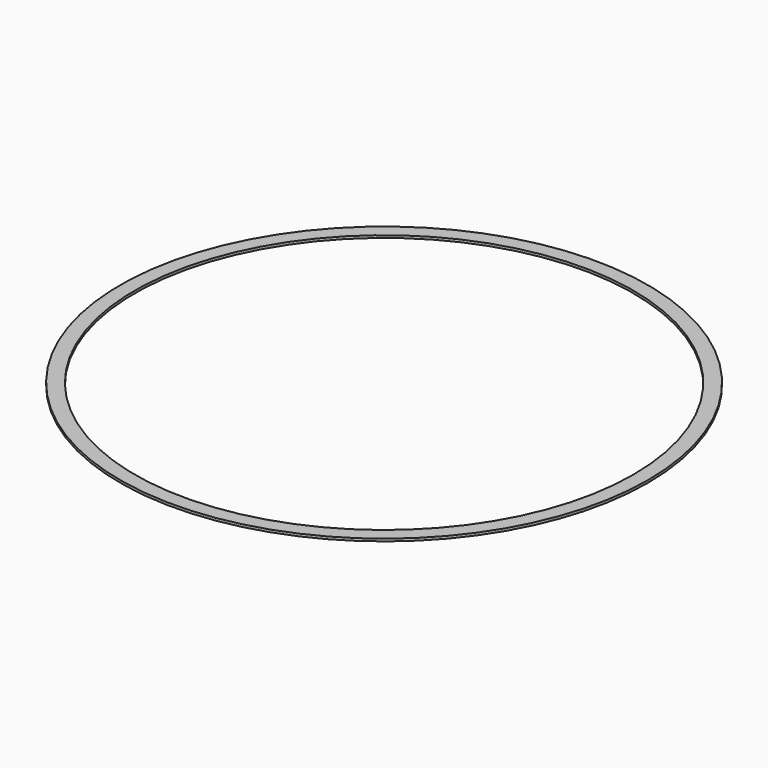
from build123d import *

# Parameters (mm, degrees)
F0_R     = 456.78598
F0_R_2   = 431.38598
F1_DEPTH = 4.2333333333


# Not quite as in the source:
# - a length typed as a fraction of an inch, garbled in the dataset ("3 / 203.2 mm" for 3/8 in), is restored


with BuildPart() as f1:
    # F0 (on Top) → F1 (new body)
    with BuildSketch(Plane.XY):
        Circle(F0_R)
        Circle(F0_R_2, mode=Mode.SUBTRACT)
    extrude(amount=F1_DEPTH)


solid = f1.part
